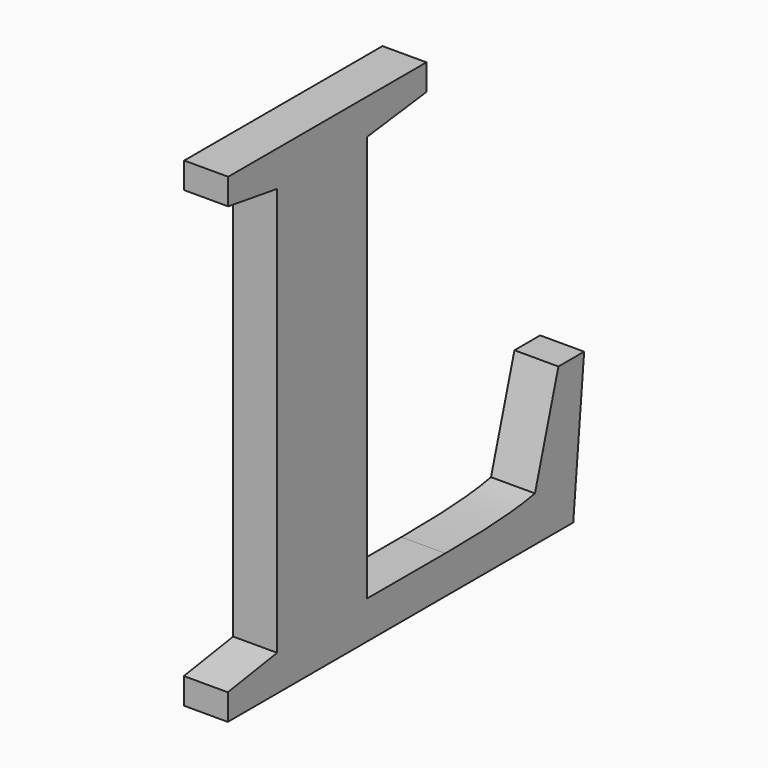
from build123d import *

# Parameters (mm, degrees)
F0_TEXT_SIZE = 635
F1_DEPTH     = 38.1


# Not quite as in the source:
# - Text() gives the source's letters only with a copy of the font that has no kerning and outlines rounded to 1/6400 em; it was checked with that copy


with BuildPart() as f1:
    # F0 (on Right) → F1 (new body)
    with BuildSketch(Plane.YZ):
        with Locations((-436.5625, 0)):
            Text('L', F0_TEXT_SIZE, font='Tinos', font_style=FontStyle.BOLD, text_align=(TextAlign.LEFT, TextAlign.BOTTOM))
    extrude(amount=F1_DEPTH)


solid = f1.part
